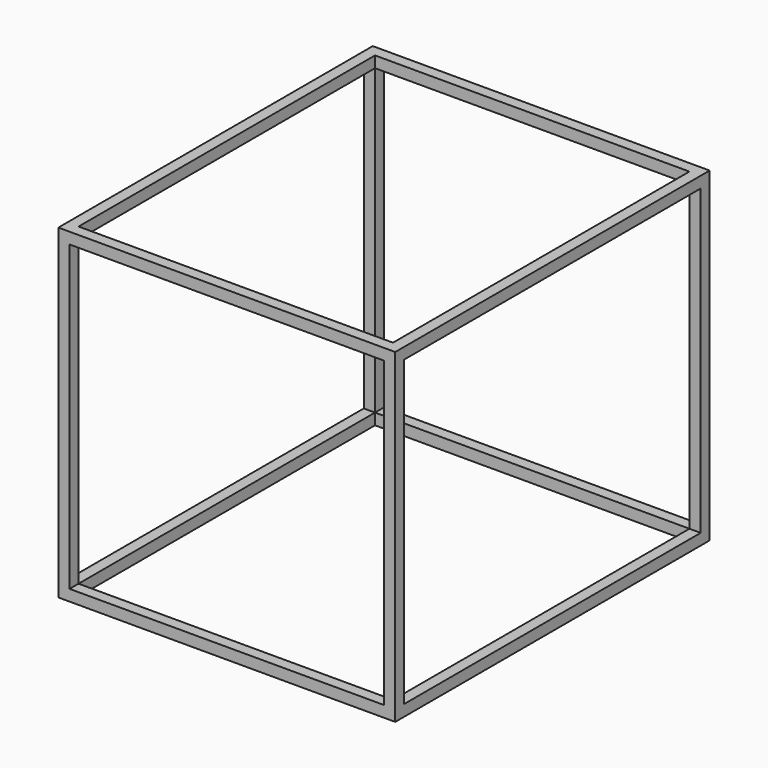
from build123d import *

# Parameters (mm, degrees)
F0_W      = 20
F0_H      = 660
F0_H_2    = 20
F1_DEPTH  = 20
F2_DEPTH  = 580
F3_W      = 20
F3_H      = 20
F4_DEPTH  = 660
F5_W      = 20
F5_H      = 20
F6_DEPTH  = 560
F7_W      = 20
F7_H      = 20
F8_DEPTH  = 560
F9_W      = 20
F9_H      = 20
F10_DEPTH = 660


# Not quite as in the source:
# - a feature names something its author has since deleted; it is built from what else it names


with BuildPart() as f1:
    # F0 (on Top) → F1 (new body)
    with BuildSketch(Plane.XY):
        Polygon((250.936165452, 480.5163520575), (-329.063834548, 480.5163520575), (-329.063834548, 460.5163520575), (230.936165452, 460.5163520575), (230.936165452, -199.4836479425), (-329.063834548, -199.4836479425), (-329.063834548, -219.4836479425), (250.936165452, -219.4836479425), align=None)
        with Locations((-339.063834548, 130.5163520575)):
            Rectangle(F0_W, F0_H)
        with Locations((-339.063834548, 470.5163520575)):
            Rectangle(F0_W, F0_H_2)
        with Locations((-339.063834548, -209.4836479425)):
            Rectangle(F0_W, F0_H_2)
    extrude(amount=F1_DEPTH)

    # F0 (on Top) → F2 (join)
    with BuildSketch(Plane.XY):
        with Locations((-339.063834548, 470.5163520575)):
            Rectangle(F0_W, F0_H_2)
        with Locations((-339.063834548, -209.4836479425)):
            Rectangle(F0_W, F0_H_2)
    extrude(amount=F2_DEPTH)

    # F3 (on face) → F4 (join)
    with BuildSketch(Plane(origin=(0, -199.4836479425, 0), x_dir=(-1, 0, 0), z_dir=(0, 1, 0))):
        with Locations((339.063834548, 570)):
            Rectangle(F3_W, F3_H)
    extrude(amount=F4_DEPTH)

    # F5 (on face) → F6 (join)
    with BuildSketch(Plane.YZ.offset(-329.063834548)):
        with Locations((-209.4836479425, 570)):
            Rectangle(F5_W, F5_H)
        with Locations((470.5163520575, 570)):
            Rectangle(F5_W, F5_H)
    extrude(amount=F6_DEPTH)

    # F7 (on face) → F8 (join)
    with BuildSketch(Plane.XY.offset(20)):
        with Locations((240.936165452, 470.5163520575)):
            Rectangle(F7_W, F7_H)
        with Locations((240.936165452, -209.4836479425)):
            Rectangle(F7_W, F7_H)
    extrude(amount=F8_DEPTH)

    # F9 (on face) → F10 (join)
    with BuildSketch(Plane.XZ.offset(-460.5163520575)):
        with Locations((240.936165452, 570)):
            Rectangle(F9_W, F9_H)
    extrude(amount=F10_DEPTH)


solid = f1.part
